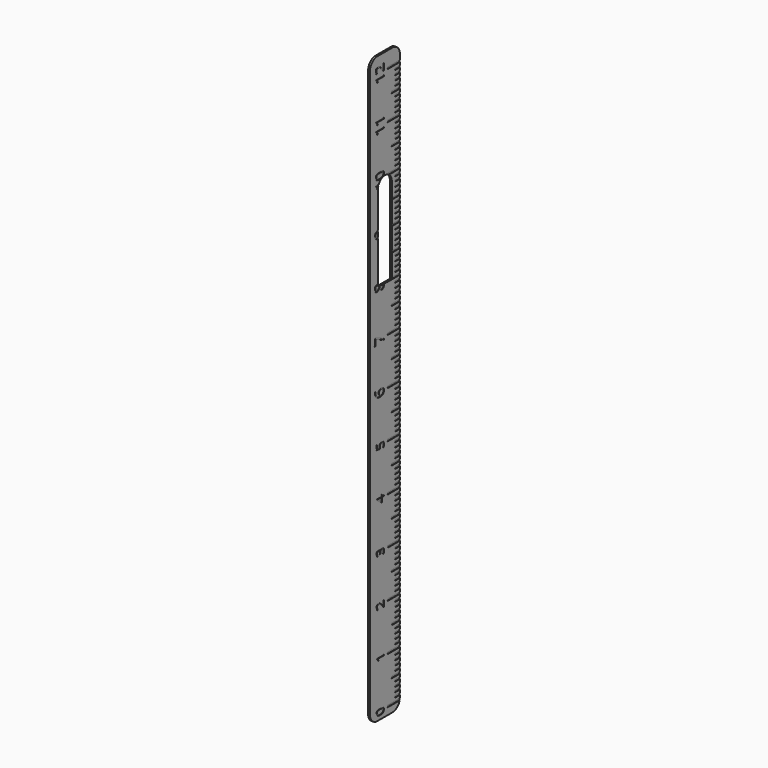
from build123d import *

# Parameters (mm, degrees)
F0_W           = 10
F0_H           = 160
F1_DEPTH       = 0.1
F2_W           = 4
F2_H           = 0.4
F2_W_2         = 3
F2_W_3         = 2
F2_TEXT_SIZE   = 2.7777777778
F2_TEXT_SIZE_2 = 3.4258994799
F2_TEXT_SIZE_3 = 3.0868508472
F3_DEPTH       = 5
F4_W           = 8
F4_H           = 125
F5_DEPTH       = 0.4
F6_R           = 2
F8_DEPTH       = 12.5
F10_W          = 25.6892092228
F10_H          = 35.3538990021
F10_W_2        = 17.939006567
F11_DEPTH      = 12.5


# Not quite as in the source:
# - Text() gives the source's letters only with a copy of the font that has no kerning and outlines rounded to 1/6400 em; it was checked with that copy


with BuildPart() as f1:
    # F0 (on Right) → F1 (new body)
    with BuildSketch(Plane.YZ):
        with Locations((-15, 80)):
            Rectangle(F0_W, F0_H)
    extrude(amount=F1_DEPTH)

    # F2 (on Right) → F3 (join, symmetric)
    with BuildSketch(Plane.YZ):
        with Locations((-12, 10.2)):
            Rectangle(F2_W, F2_H)
        with Locations((-12, 20.2)):
            Rectangle(F2_W, F2_H)
        with Locations((-12, 30.2)):
            Rectangle(F2_W, F2_H)
        with Locations((-12, 40.2)):
            Rectangle(F2_W, F2_H)
        with Locations((-12, 50.2)):
            Rectangle(F2_W, F2_H)
        with Locations((-12, 60.2)):
            Rectangle(F2_W, F2_H)
        with Locations((-12, 70.2)):
            Rectangle(F2_W, F2_H)
        with Locations((-12, 80.2)):
            Rectangle(F2_W, F2_H)
        with Locations((-12, 90.2)):
            Rectangle(F2_W, F2_H)
        with Locations((-12, 100.2)):
            Rectangle(F2_W, F2_H)
        with Locations((-12, 110.2)):
            Rectangle(F2_W, F2_H)
        with Locations((-12, 120.2)):
            Rectangle(F2_W, F2_H)
        with Locations((-12, 130.2)):
            Rectangle(F2_W, F2_H)
        with Locations((-12, 140.2)):
            Rectangle(F2_W, F2_H)
        with Locations((-11.5, 15.2)):
            Rectangle(F2_W_2, F2_H)
        with Locations((-11, 11.2)):
            Rectangle(F2_W_3, F2_H)
        with Locations((-11, 12.2)):
            Rectangle(F2_W_3, F2_H)
        with Locations((-11, 13.2)):
            Rectangle(F2_W_3, F2_H)
        with Locations((-11, 14.2)):
            Rectangle(F2_W_3, F2_H)
        with Locations((-11, 16.2)):
            Rectangle(F2_W_3, F2_H)
        with Locations((-11, 17.2)):
            Rectangle(F2_W_3, F2_H)
        with Locations((-11, 18.2)):
            Rectangle(F2_W_3, F2_H)
        with Locations((-11, 19.2)):
            Rectangle(F2_W_3, F2_H)
        with Locations((-11, 22.2)):
            Rectangle(F2_W_3, F2_H)
        with Locations((-11, 21.2)):
            Rectangle(F2_W_3, F2_H)
        with Locations((-11, 23.2)):
            Rectangle(F2_W_3, F2_H)
        with Locations((-11, 28.2)):
            Rectangle(F2_W_3, F2_H)
        with Locations((-11.5, 25.2)):
            Rectangle(F2_W_2, F2_H)
        with Locations((-11, 29.2)):
            Rectangle(F2_W_3, F2_H)
        with Locations((-11, 24.2)):
            Rectangle(F2_W_3, F2_H)
        with Locations((-11, 26.2)):
            Rectangle(F2_W_3, F2_H)
        with Locations((-11, 27.2)):
            Rectangle(F2_W_3, F2_H)
        with Locations((-11, 32.2)):
            Rectangle(F2_W_3, F2_H)
        with Locations((-11, 31.2)):
            Rectangle(F2_W_3, F2_H)
        with Locations((-11, 33.2)):
            Rectangle(F2_W_3, F2_H)
        with Locations((-11, 38.2)):
            Rectangle(F2_W_3, F2_H)
        with Locations((-11.5, 35.2)):
            Rectangle(F2_W_2, F2_H)
        with Locations((-11, 39.2)):
            Rectangle(F2_W_3, F2_H)
        with Locations((-11, 34.2)):
            Rectangle(F2_W_3, F2_H)
        with Locations((-11, 36.2)):
            Rectangle(F2_W_3, F2_H)
        with Locations((-11, 37.2)):
            Rectangle(F2_W_3, F2_H)
        with Locations((-11, 42.2)):
            Rectangle(F2_W_3, F2_H)
        with Locations((-11, 41.2)):
            Rectangle(F2_W_3, F2_H)
        with Locations((-11, 43.2)):
            Rectangle(F2_W_3, F2_H)
        with Locations((-11, 48.2)):
            Rectangle(F2_W_3, F2_H)
        with Locations((-11.5, 45.2)):
            Rectangle(F2_W_2, F2_H)
        with Locations((-11, 49.2)):
            Rectangle(F2_W_3, F2_H)
        with Locations((-11, 44.2)):
            Rectangle(F2_W_3, F2_H)
        with Locations((-11, 46.2)):
            Rectangle(F2_W_3, F2_H)
        with Locations((-11, 47.2)):
            Rectangle(F2_W_3, F2_H)
        with Locations((-11, 52.2)):
            Rectangle(F2_W_3, F2_H)
        with Locations((-11, 51.2)):
            Rectangle(F2_W_3, F2_H)
        with Locations((-11, 53.2)):
            Rectangle(F2_W_3, F2_H)
        with Locations((-11, 58.2)):
            Rectangle(F2_W_3, F2_H)
        with Locations((-11.5, 55.2)):
            Rectangle(F2_W_2, F2_H)
        with Locations((-11, 59.2)):
            Rectangle(F2_W_3, F2_H)
        with Locations((-11, 54.2)):
            Rectangle(F2_W_3, F2_H)
        with Locations((-11, 56.2)):
            Rectangle(F2_W_3, F2_H)
        with Locations((-11, 57.2)):
            Rectangle(F2_W_3, F2_H)
        with Locations((-11, 62.2)):
            Rectangle(F2_W_3, F2_H)
        with Locations((-11, 61.2)):
            Rectangle(F2_W_3, F2_H)
        with Locations((-11, 63.2)):
            Rectangle(F2_W_3, F2_H)
        with Locations((-11, 68.2)):
            Rectangle(F2_W_3, F2_H)
        with Locations((-11.5, 65.2)):
            Rectangle(F2_W_2, F2_H)
        with Locations((-11, 69.2)):
            Rectangle(F2_W_3, F2_H)
        with Locations((-11, 64.2)):
            Rectangle(F2_W_3, F2_H)
        with Locations((-11, 66.2)):
            Rectangle(F2_W_3, F2_H)
        with Locations((-11, 67.2)):
            Rectangle(F2_W_3, F2_H)
        with Locations((-11, 72.2)):
            Rectangle(F2_W_3, F2_H)
        with Locations((-11, 71.2)):
            Rectangle(F2_W_3, F2_H)
        with Locations((-11, 73.2)):
            Rectangle(F2_W_3, F2_H)
        with Locations((-11, 78.2)):
            Rectangle(F2_W_3, F2_H)
        with Locations((-11.5, 75.2)):
            Rectangle(F2_W_2, F2_H)
        with Locations((-11, 79.2)):
            Rectangle(F2_W_3, F2_H)
        with Locations((-11, 74.2)):
            Rectangle(F2_W_3, F2_H)
        with Locations((-11, 76.2)):
            Rectangle(F2_W_3, F2_H)
        with Locations((-11, 77.2)):
            Rectangle(F2_W_3, F2_H)
        with Locations((-11, 82.2)):
            Rectangle(F2_W_3, F2_H)
        with Locations((-11, 81.2)):
            Rectangle(F2_W_3, F2_H)
        with Locations((-11, 83.2)):
            Rectangle(F2_W_3, F2_H)
        with Locations((-11, 88.2)):
            Rectangle(F2_W_3, F2_H)
        with Locations((-11.5, 85.2)):
            Rectangle(F2_W_2, F2_H)
        with Locations((-11, 89.2)):
            Rectangle(F2_W_3, F2_H)
        with Locations((-11, 84.2)):
            Rectangle(F2_W_3, F2_H)
        with Locations((-11, 86.2)):
            Rectangle(F2_W_3, F2_H)
        with Locations((-11, 87.2)):
            Rectangle(F2_W_3, F2_H)
        with Locations((-11, 92.2)):
            Rectangle(F2_W_3, F2_H)
        with Locations((-11, 91.2)):
            Rectangle(F2_W_3, F2_H)
        with Locations((-11, 93.2)):
            Rectangle(F2_W_3, F2_H)
        with Locations((-11, 98.2)):
            Rectangle(F2_W_3, F2_H)
        with Locations((-11.5, 95.2)):
            Rectangle(F2_W_2, F2_H)
        with Locations((-11, 99.2)):
            Rectangle(F2_W_3, F2_H)
        with Locations((-11, 94.2)):
            Rectangle(F2_W_3, F2_H)
        with Locations((-11, 96.2)):
            Rectangle(F2_W_3, F2_H)
        with Locations((-11, 97.2)):
            Rectangle(F2_W_3, F2_H)
        with Locations((-11, 102.2)):
            Rectangle(F2_W_3, F2_H)
        with Locations((-11, 101.2)):
            Rectangle(F2_W_3, F2_H)
        with Locations((-11, 103.2)):
            Rectangle(F2_W_3, F2_H)
        with Locations((-11, 108.2)):
            Rectangle(F2_W_3, F2_H)
        with Locations((-11.5, 105.2)):
            Rectangle(F2_W_2, F2_H)
        with Locations((-11, 109.2)):
            Rectangle(F2_W_3, F2_H)
        with Locations((-11, 104.2)):
            Rectangle(F2_W_3, F2_H)
        with Locations((-11, 106.2)):
            Rectangle(F2_W_3, F2_H)
        with Locations((-11, 107.2)):
            Rectangle(F2_W_3, F2_H)
        with Locations((-11, 112.2)):
            Rectangle(F2_W_3, F2_H)
        with Locations((-11, 111.2)):
            Rectangle(F2_W_3, F2_H)
        with Locations((-11, 113.2)):
            Rectangle(F2_W_3, F2_H)
        with Locations((-11, 118.2)):
            Rectangle(F2_W_3, F2_H)
        with Locations((-11.5, 115.2)):
            Rectangle(F2_W_2, F2_H)
        with Locations((-11, 119.2)):
            Rectangle(F2_W_3, F2_H)
        with Locations((-11, 114.2)):
            Rectangle(F2_W_3, F2_H)
        with Locations((-11, 116.2)):
            Rectangle(F2_W_3, F2_H)
        with Locations((-11, 117.2)):
            Rectangle(F2_W_3, F2_H)
        with Locations((-11, 122.2)):
            Rectangle(F2_W_3, F2_H)
        with Locations((-11, 121.2)):
            Rectangle(F2_W_3, F2_H)
        with Locations((-11, 123.2)):
            Rectangle(F2_W_3, F2_H)
        with Locations((-11, 128.2)):
            Rectangle(F2_W_3, F2_H)
        with Locations((-11.5, 125.2)):
            Rectangle(F2_W_2, F2_H)
        with Locations((-11, 129.2)):
            Rectangle(F2_W_3, F2_H)
        with Locations((-11, 124.2)):
            Rectangle(F2_W_3, F2_H)
        with Locations((-11, 126.2)):
            Rectangle(F2_W_3, F2_H)
        with Locations((-11, 127.2)):
            Rectangle(F2_W_3, F2_H)
        with Locations((-11, 132.2)):
            Rectangle(F2_W_3, F2_H)
        with Locations((-11, 131.2)):
            Rectangle(F2_W_3, F2_H)
        with Locations((-11, 133.2)):
            Rectangle(F2_W_3, F2_H)
        with Locations((-11, 138.2)):
            Rectangle(F2_W_3, F2_H)
        with Locations((-11.5, 135.2)):
            Rectangle(F2_W_2, F2_H)
        with Locations((-11, 139.2)):
            Rectangle(F2_W_3, F2_H)
        with Locations((-11, 134.2)):
            Rectangle(F2_W_3, F2_H)
        with Locations((-11, 136.2)):
            Rectangle(F2_W_3, F2_H)
        with Locations((-11, 137.2)):
            Rectangle(F2_W_3, F2_H)
        with Locations(Location((-17, 10.8151041667), (0, 0, -90))):
            Text('0', F2_TEXT_SIZE, font='Open Sans', text_align=(TextAlign.LEFT, TextAlign.BOTTOM))
        with Locations(Location((-15, 19.4251302083), (0, 0, 90))):
            Text('1', F2_TEXT_SIZE, font='Open Sans', text_align=(TextAlign.LEFT, TextAlign.BOTTOM))
        with Locations(Location((-15, 29.1903211806), (0, 0, 90))):
            Text('2', F2_TEXT_SIZE, font='Open Sans', text_align=(TextAlign.LEFT, TextAlign.BOTTOM))
        with Locations(Location((-15, 39.197265625), (0, 0, 90))):
            Text('3', F2_TEXT_SIZE, font='Open Sans', text_align=(TextAlign.LEFT, TextAlign.BOTTOM))
        with Locations(Location((-15, 49.1436631944), (0, 0, 90))):
            Text('4', F2_TEXT_SIZE, font='Open Sans', text_align=(TextAlign.LEFT, TextAlign.BOTTOM))
        with Locations(Location((-15, 59.1957465278), (0, 0, 90))):
            Text('5', F2_TEXT_SIZE, font='Open Sans', text_align=(TextAlign.LEFT, TextAlign.BOTTOM))
        with Locations(Location((-15, 68.993106731), (0, 0, 90))):
            Text('6', F2_TEXT_SIZE_2, font='Open Sans', text_align=(TextAlign.LEFT, TextAlign.BOTTOM))
        with Locations(Location((-15, 78.9965861602), (0, 0, 90))):
            Text('7', F2_TEXT_SIZE_2, font='Open Sans', text_align=(TextAlign.LEFT, TextAlign.BOTTOM))
        with Locations(Location((-15, 88.9981920505), (0, 0, 90))):
            Text('8', F2_TEXT_SIZE_2, font='Open Sans', text_align=(TextAlign.LEFT, TextAlign.BOTTOM))
        with Locations(Location((-15, 99.0014038313), (0, 0, 90))):
            Text('9', F2_TEXT_SIZE_2, font='Open Sans', text_align=(TextAlign.LEFT, TextAlign.BOTTOM))
        with Locations(Location((-15, 108.2117969506), (0, 0, 90))):
            Text('10', F2_TEXT_SIZE_3, font='Open Sans', text_align=(TextAlign.LEFT, TextAlign.BOTTOM))
        with Locations(Location((-15, 118.4787613169), (0, 0, 90))):
            Text('11', F2_TEXT_SIZE_3, font='Open Sans', text_align=(TextAlign.LEFT, TextAlign.BOTTOM))
        with Locations(Location((-15, 128.2178259562), (0, 0, 90))):
            Text('12', F2_TEXT_SIZE_3, font='Open Sans', text_align=(TextAlign.LEFT, TextAlign.BOTTOM))
        with Locations(Location((-15, 138.2255430833), (0, 0, 90))):
            Text('13', F2_TEXT_SIZE_3, font='Open Sans', text_align=(TextAlign.LEFT, TextAlign.BOTTOM))
    extrude(amount=F3_DEPTH, both=True)


with BuildPart() as f5:
    # F4 (on Right) → F5 (new body)
    with BuildSketch(Plane.YZ):
        with Locations((30.2877472714, 96.0264432559)):
            Rectangle(F4_W, F4_H)
    extrude(amount=F5_DEPTH)

    # F6
    f6_edges = [f5.edges().sort_by_distance(p)[0] for p in [
        (0.2, 26.287747, 158.526443),
        (0.2, 34.287747, 158.526443),
        (0.2, 34.287747, 33.526443),
        (0.2, 26.287747, 33.526443),
    ]]
    fillet(f6_edges, radius=F6_R)

    # F7 (on face) → F8 (cut, symmetric)
    with BuildSketch(Plane.YZ.offset(0.4)):
        with BuildLine():
            Line((28.4577472714, 133.5264432559), (28.4577472714, 115.0264432559))
            Line((28.4577472714, 115.0264432559), (32.1177472714, 115.0264432559))
            Line((32.1177472714, 115.0264432559), (32.1177472714, 133.5264432559))
            ThreePointArc((32.1177472714, 133.5264432559), (30.2877472714, 135.3564432559), (28.4577472714, 133.5264432559))
        make_face()
    extrude(amount=F8_DEPTH, both=True, mode=Mode.SUBTRACT)


with BuildPart() as f1_1:
    # F9: moved
    add(f1.part.moved(Location((5.3, 45, 25))))

    # F10 (on face) → F11 (cut, symmetric)
    with BuildSketch(Plane.YZ.offset(5.4)):
        with Locations((19.1553953886, 175.4610091448)):
            Rectangle(F10_W, F10_H)
        Polygon((32, 196.6169327497), (32, 193.1379586458), (49.939006567, 193.1379586458), (49.939006567, 157.7840596437), (32, 157.7840596437), (32, 155.9), (54.170191288, 155.9), (54.170191288, 196.6169327497), align=None)
        with Locations((40.9695032835, 175.4610091448)):
            Rectangle(F10_W_2, F10_H)
    extrude(amount=F11_DEPTH, both=True, mode=Mode.SUBTRACT)


with BuildPart() as f5_1:
    add(f5.part)

    # F12: cut F1
    add(f1_1.part, mode=Mode.SUBTRACT)


solid = f5_1.part
